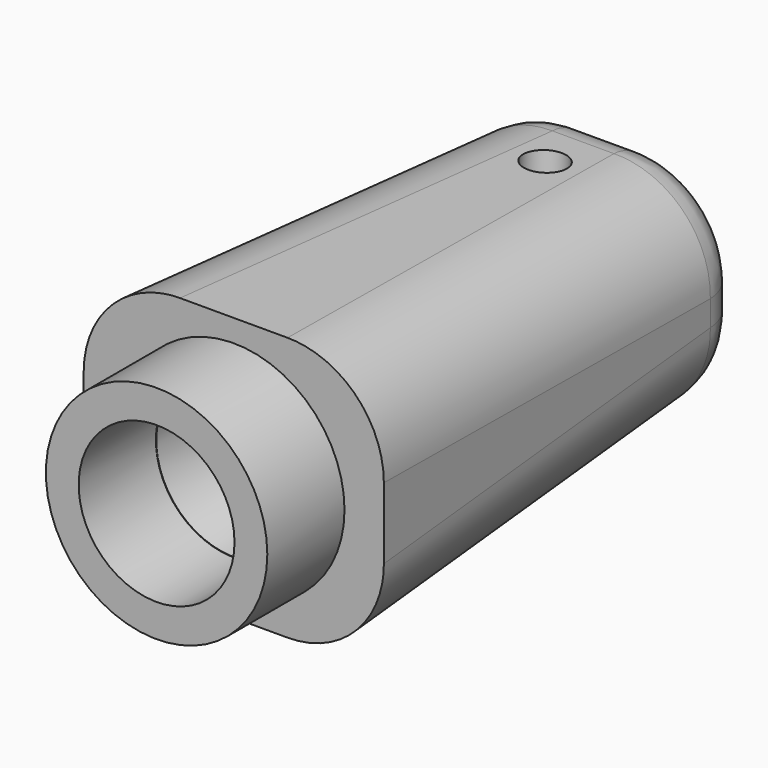
from build123d import *

# Parameters (mm, degrees)
F0_W                   = 65.7132863998
F0_H                   = 56.1922863126
F1_DEPTH               = 127
DRAFT_F1_DRAFTED_ANGLE = -3
F2_R                   = 25.4
F3_R                   = 20.4053446834
F4_DEPTH               = 114.3
F4_TAPER               = 3
F5_R                   = 5.5034244633
F6_DEPTH               = 76.2
F7_R                   = 12.7
F8_R                   = 29.1486000132
F8_R_2                 = 20.5124746621
F9_DEPTH               = 25.4


# Not quite as in the source:
# - an extrude with a draft is written as a straight extrude whose walls are then drafted


with BuildPart() as f1:
    # F0 (on Front) → F1 (new body)
    with BuildSketch(Plane.XZ):
        with Locations((-111.430555582, 28.0961431563)):
            Rectangle(F0_W, F0_H)
    extrude(amount=F1_DEPTH)

    # draft_F1_drafted
    draft_f1_drafted_walls = [f1.faces().sort_by_distance(p)[0] for p in [
        (-111.430555582, -84.6666666667, 0),
        (-78.5739123821, -84.6666666667, 28.0961431563),
        (-111.430555582, -84.6666666667, 56.1922863126),
        (-144.287198782, -84.6666666667, 28.0961431563),
    ]]
    draft(draft_f1_drafted_walls, neutral_plane=Plane.XZ, angle=DRAFT_F1_DRAFTED_ANGLE)

    # F2
    f2_edges = [f1.edges().sort_by_distance(p)[0] for p in [
        (-147.615093, -63.5, -3.327894),
        (-75.246018, -63.5, -3.327894),
        (-75.246018, -63.5, 59.52018),
        (-147.615093, -63.5, 59.52018),
    ]]
    fillet(f2_edges, radius=F2_R)

    # F3 (on face) → F4 (cut)
    with BuildSketch(Plane.XZ.offset(127)):
        with Locations((-111.430555582, 27.8455689549)):
            Circle(F3_R)
    extrude(amount=-F4_DEPTH, taper=F4_TAPER, mode=Mode.SUBTRACT)

    # F5 (on face) → F6 (cut)
    with BuildSketch(Plane(origin=(0, 2.9368466679, 56.0383727006), x_dir=(1, 0, 0), z_dir=(0, 0.0523359562, 0.9986295348))):
        with Locations((-111.430555582, -27.5344327092)):
            Circle(F5_R)
    extrude(amount=-F6_DEPTH, mode=Mode.SUBTRACT)

    # F7
    f7_edges = [f1.edges().sort_by_distance(p)[0] for p in [
        (-111.430556, 0, 0),
        (-136.862116, 0, 7.425083),
        (-85.998995, 0, 7.425083),
        (-144.287199, 0, 28.096143),
        (-78.573912, 0, 28.096143),
        (-136.862116, 0, 48.767203),
        (-85.998995, 0, 48.767203),
        (-111.430556, 0, 56.192286),
    ]]
    fillet(f7_edges, radius=F7_R)

    # F8 (on face) → F9 (join)
    with BuildSketch(Plane.XZ.offset(127)):
        with Locations((-111.430555582, 27.8455689549)):
            Circle(F8_R)
        with Locations((-111.430555582, 27.8455689549)):
            Circle(F8_R_2, mode=Mode.SUBTRACT)
    extrude(amount=F9_DEPTH)


solid = f1.part
